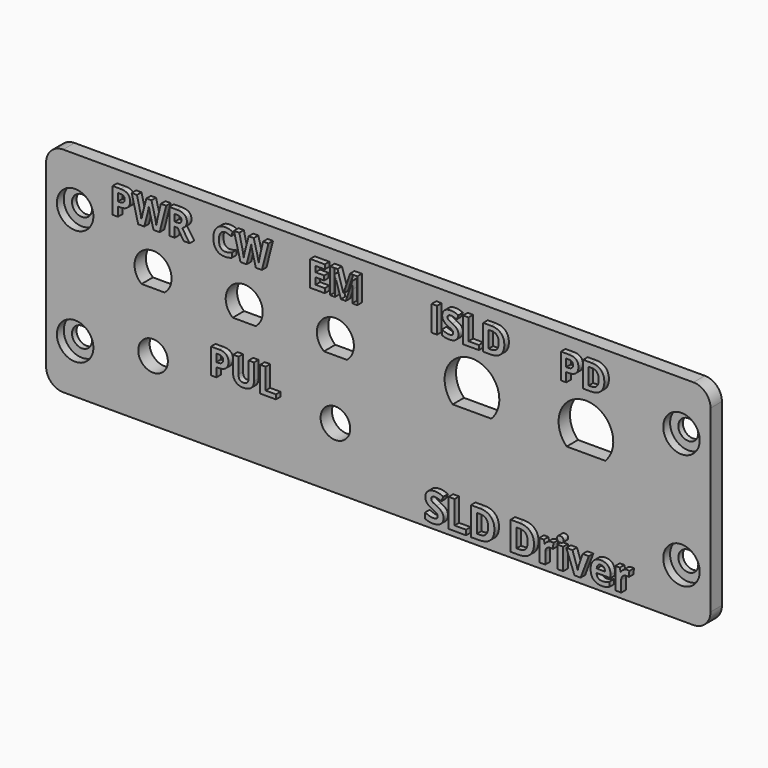
from build123d import *

# Parameters (mm, degrees)
F0_R          = 1.75
F1_DEPTH      = 2.5
F2_R          = 3.2
F3_DEPTH      = 1.5
F4_W          = 2.5
F4_H          = 6
F5_DEPTH      = 1.25
F6_R          = 2.6
F7_DEPTH      = 2.501
F8_TEXT_SIZE  = 6.25
F9_DEPTH      = 1
F10_TEXT_SIZE = 6.25
F11_DEPTH     = 1
F12_TEXT_SIZE = 6.9444444444
F13_DEPTH     = 1


# Not quite as in the source:
# - Text() gives the source's letters only with a copy of the font that has no kerning and outlines rounded to 1/6400 em; it was checked with that copy


with BuildPart() as f1:
    # F0 (on Front) → F1 (new body)
    with BuildSketch(Plane.XZ):
        with BuildLine():
            Line((55.3, 18.75), (-55.3, 18.75))
            ThreePointArc((-55.3, 18.75), (-57.4213203436, 17.8713203436), (-58.3, 15.75))
            Line((-58.3, 15.75), (-58.3, -15.75))
            ThreePointArc((-58.3, -15.75), (-57.4213203436, -17.8713203436), (-55.3, -18.75))
            Line((-55.3, -18.75), (55.3, -18.75))
            ThreePointArc((55.3, -18.75), (57.4213203436, -17.8713203436), (58.3, -15.75))
            Line((58.3, -15.75), (58.3, 15.75))
            ThreePointArc((58.3, 15.75), (57.4213203436, 17.8713203436), (55.3, 18.75))
        make_face()
        with Locations((-53.2, -10.15)):
            Circle(F0_R, mode=Mode.SUBTRACT)
        with Locations((53.2, -10.15)):
            Circle(F0_R, mode=Mode.SUBTRACT)
        with Locations((-53.2, 10.15)):
            Circle(F0_R, mode=Mode.SUBTRACT)
        with Locations((53.2, 10.15)):
            Circle(F0_R, mode=Mode.SUBTRACT)
    extrude(amount=F1_DEPTH)

    # F2 (on face) → F3 (cut)
    with BuildSketch(Plane.XZ.offset(2.5)):
        with Locations((-53.2, 10.15)):
            Circle(F2_R)
        with Locations((53.2, 10.15)):
            Circle(F2_R)
        with Locations((-53.2, -10.15)):
            Circle(F2_R)
        with Locations((53.2, -10.15)):
            Circle(F2_R)
    extrude(amount=-F3_DEPTH, mode=Mode.SUBTRACT)

    # F4 (on face) → F5 (cut)
    with BuildSketch(Plane(origin=(0, 0, 0), x_dir=(-1, 0, 0), z_dir=(0, 1, 0))):
        with Locations((57.05, 0)):
            Rectangle(F4_W, F4_H)
    extrude(amount=-F5_DEPTH, mode=Mode.SUBTRACT)

    # F6 (on face) → F7 (cut, through all)
    with BuildSketch(Plane.XZ.offset(2.5)):
        with BuildLine():
            Line((-41.5450463315, 2.45), (-37.5151579956, 2.45))
            ThreePointArc((-37.5151579956, 2.45), (-39.5301021636, 8.25), (-41.5450463315, 2.45))
        make_face()
        with BuildLine():
            Line((-25.5450463315, 2.45), (-21.5151579956, 2.45))
            ThreePointArc((-21.5151579956, 2.45), (-23.5301021636, 8.25), (-25.5450463315, 2.45))
        make_face()
        with BuildLine():
            Line((-9.5450463315, 2.45), (-5.5151579956, 2.45))
            ThreePointArc((-5.5151579956, 2.45), (-7.5301021636, 8.25), (-9.5450463315, 2.45))
        make_face()
        with BuildLine():
            Line((33.0481012037, 1.6), (39.8245309422, 1.6))
            ThreePointArc((39.8245309422, 1.6), (36.4363160729, 9.8), (33.0481012037, 1.6))
        make_face()
        with BuildLine():
            Line((13.0481012037, 1.6), (19.8245309422, 1.6))
            ThreePointArc((19.8245309422, 1.6), (16.4363160729, 9.8), (13.0481012037, 1.6))
        make_face()
        with Locations((-39.5301021636, -8)):
            Circle(F6_R)
        with Locations((-7.5301021636, -8)):
            Circle(F6_R)
    extrude(amount=-F7_DEPTH, mode=Mode.SUBTRACT)

    # F8 (on face) → F9 (join)
    with BuildSketch(Plane.XZ.offset(2.5)):
        with Locations((-46.4006096217, 12.147965841)):
            Text('PWR', F8_TEXT_SIZE, font='Open Sans', font_style=FontStyle.BOLD, text_align=(TextAlign.LEFT, TextAlign.BOTTOM))
        with Locations((-28.5068553936, 12.147965841)):
            Text('CW', F8_TEXT_SIZE, font='Open Sans', font_style=FontStyle.BOLD, text_align=(TextAlign.LEFT, TextAlign.BOTTOM))
        with Locations((-11.7175406776, 12.147965841)):
            Text('EM', F8_TEXT_SIZE, font='Open Sans', font_style=FontStyle.BOLD, text_align=(TextAlign.LEFT, TextAlign.BOTTOM))
        with Locations((9.6073653549, 12.147965841)):
            Text('ISLD', F8_TEXT_SIZE, font='Open Sans', font_style=FontStyle.BOLD, text_align=(TextAlign.LEFT, TextAlign.BOTTOM))
        with Locations((32.2735868394, 12.147965841)):
            Text('PD', F8_TEXT_SIZE, font='Open Sans', font_style=FontStyle.BOLD, text_align=(TextAlign.LEFT, TextAlign.BOTTOM))
    extrude(amount=F9_DEPTH)

    # F10 (on face) → F11 (join)
    with BuildSketch(Plane.XZ.offset(2.5)):
        with Locations((-29.1328607675, -7.0470169045)):
            Text('PUL', F10_TEXT_SIZE, font='Open Sans', font_style=FontStyle.BOLD, text_align=(TextAlign.LEFT, TextAlign.BOTTOM))
    extrude(amount=F11_DEPTH)

    # F12 (on face) → F13 (join)
    with BuildSketch(Plane.XZ.offset(2.5)):
        with Locations((8.6862881064, -17.1977844553)):
            Text('SLD Driver', F12_TEXT_SIZE, font='Open Sans', font_style=FontStyle.BOLD, text_align=(TextAlign.LEFT, TextAlign.BOTTOM))
    extrude(amount=F13_DEPTH)


solid = f1.part
